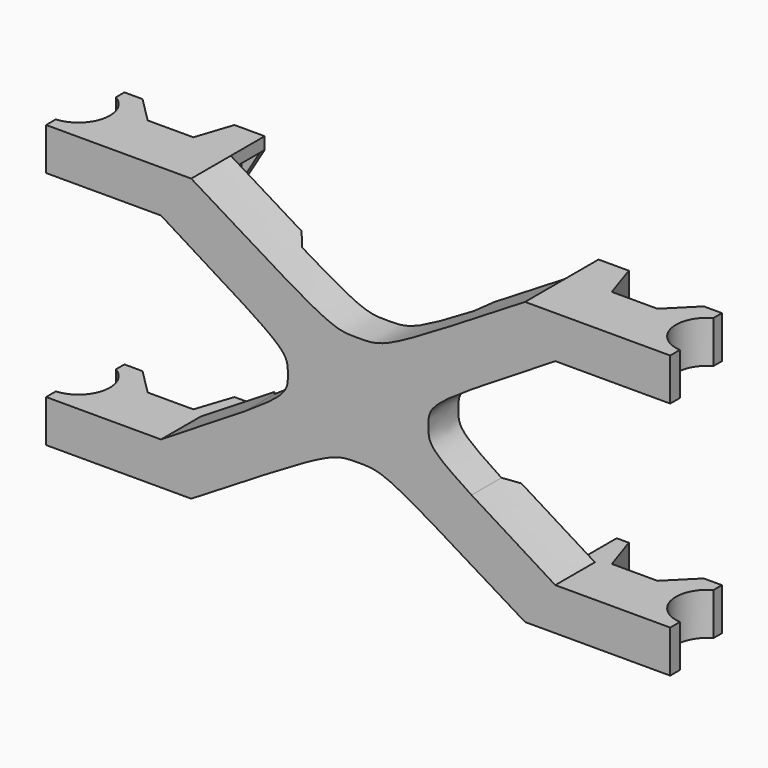
from build123d import *

# Parameters (mm, degrees)
F3_DEPTH = 25
F4_DEPTH = 15
F5_DEPTH = 3.5
F6_DEPTH = 4.5
F7_SIZE  = 0.99999
F8_DEPTH = 0.5


# Not quite as in the source:
# - a fillet or chamfer is up to 0.001 mm smaller than in the source, because OpenCascade refuses the exact size


with BuildPart() as f3:
    # F1 (on Front) → F3 (new body)
    with BuildSketch(Plane.XZ):
        Polygon((-13.8, 10.65), (-13.8, 11.65), (-27.9639077127, 11.65), (-27.9639077127, 8.15), (-16.3, 8.15), (-15.3, 8.15), (-15.3, 10.65), align=None)
        Polygon((-15.3, 8.15), (-13.8, 10.65), (-15.3, 10.65), align=None)
        with BuildLine():
            add(Edge.make_bspline(
                [(-13.8, 11.65), (-10.9198868997, 9.8796682436), (-8.756331306, 8.5497860338), (-7.0968113587, 7.5507717612)],
                knots=[0, 0, 0, 0, 3.862913837, 3.862913837, 3.862913837, 3.862913837], degree=3))
            Line((-13.8, 11.65), (-13.8, 10.65))
            Line((-13.8, 10.65), (-15.3, 8.15))
            Line((-15.3, 8.15), (-16.3, 8.15))
            add(Edge.make_bspline(
                [(-16.3, 8.15), (-13.129513862, 6.2011833744), (-10.9174831538, 4.8415047533), (-9.3741615176, 3.8458017731)],
                knots=[0, 0, 0, 0, 4.015251308, 4.015251308, 4.015251308, 4.015251308], degree=3))
            Line((-9.3741615176, 3.8458017731), (-7.0968113587, 7.5507717612))
        make_face()
        with BuildLine():
            add(Edge.make_bspline(
                [(-7.0968113587, 7.5507717612), (-2.0860988453, 4.5343733594), (-1.6704895359, 4.5343733594), (0, 4.5343733594)],
                knots=[3.862913837, 3.862913837, 3.862913837, 3.862913837, 15.5264980755, 15.5264980755, 15.5264980755, 15.5264980755], degree=3))
            Line((-7.0968113587, 7.5507717612), (-9.3741615176, 3.8458017731))
            add(Edge.make_bspline(
                [(-9.3741615176, 3.8458017731), (-5.812311122, 1.5478069994), (-5.812311122, 1.1885129773), (-5.812311122, 0)],
                knots=[4.015251308, 4.015251308, 4.015251308, 4.015251308, 13.2820976506, 13.2820976506, 13.2820976506, 13.2820976506], degree=3))
            add(Edge.make_bspline(
                [(-9.3741615176, -3.8458017731), (-5.812311122, -1.5478069994), (-5.812311122, -1.1885129773), (-5.812311122, 0)],
                knots=[4.015251308, 4.015251308, 4.015251308, 4.015251308, 13.2820976506, 13.2820976506, 13.2820976506, 13.2820976506], degree=3))
            Line((-9.3741615176, -3.8458017731), (-7.0968113587, -7.5507717612))
            add(Edge.make_bspline(
                [(-7.0968113587, -7.5507717612), (-2.0860988453, -4.5343733594), (-1.6704895359, -4.5343733594), (0, -4.5343733594)],
                knots=[3.862913837, 3.862913837, 3.862913837, 3.862913837, 15.5264980755, 15.5264980755, 15.5264980755, 15.5264980755], degree=3))
            add(Edge.make_bspline(
                [(7.0968113587, -7.5507717612), (2.0860988453, -4.5343733594), (1.6704895359, -4.5343733594), (0, -4.5343733594)],
                knots=[3.862913837, 3.862913837, 3.862913837, 3.862913837, 15.5264980755, 15.5264980755, 15.5264980755, 15.5264980755], degree=3))
            Line((7.0968113587, -7.5507717612), (9.3741615176, -3.8458017731))
            add(Edge.make_bspline(
                [(9.3741615176, -3.8458017731), (5.812311122, -1.5478069994), (5.812311122, -1.1885129773), (5.812311122, 0)],
                knots=[4.015251308, 4.015251308, 4.015251308, 4.015251308, 13.2820976506, 13.2820976506, 13.2820976506, 13.2820976506], degree=3))
            add(Edge.make_bspline(
                [(9.3741615176, 3.8458017731), (5.812311122, 1.5478069994), (5.812311122, 1.1885129773), (5.812311122, 0)],
                knots=[4.015251308, 4.015251308, 4.015251308, 4.015251308, 13.2820976506, 13.2820976506, 13.2820976506, 13.2820976506], degree=3))
            Line((9.3741615176, 3.8458017731), (7.0968113587, 7.5507717612))
            add(Edge.make_bspline(
                [(7.0968113587, 7.5507717612), (2.0860988453, 4.5343733594), (1.6704895359, 4.5343733594), (0, 4.5343733594)],
                knots=[3.862913837, 3.862913837, 3.862913837, 3.862913837, 15.5264980755, 15.5264980755, 15.5264980755, 15.5264980755], degree=3))
        make_face()
        with BuildLine():
            Line((-7.0968113587, -7.5507717612), (-9.3741615176, -3.8458017731))
            add(Edge.make_bspline(
                [(-16.3, -8.15), (-13.129513862, -6.2011833744), (-10.9174831538, -4.8415047533), (-9.3741615176, -3.8458017731)],
                knots=[0, 0, 0, 0, 4.015251308, 4.015251308, 4.015251308, 4.015251308], degree=3))
            Line((-16.3, -8.15), (-15.3, -8.15))
            Line((-15.3, -8.15), (-13.8, -10.65))
            Line((-13.8, -10.65), (-13.8, -11.65))
            add(Edge.make_bspline(
                [(-13.8, -11.65), (-10.9198868997, -9.8796682436), (-8.756331306, -8.5497860338), (-7.0968113587, -7.5507717612)],
                knots=[0, 0, 0, 0, 3.862913837, 3.862913837, 3.862913837, 3.862913837], degree=3))
        make_face()
        Polygon((-13.8, -10.65), (-15.3, -8.15), (-15.3, -10.65), align=None)
        Polygon((-15.3, -8.15), (-16.3, -8.15), (-27.9639077127, -8.15), (-27.9639077127, -11.65), (-13.8, -11.65), (-13.8, -10.65), (-15.3, -10.65), align=None)
        with BuildLine():
            add(Edge.make_bspline(
                [(16.3, -8.15), (13.129513862, -6.2011833744), (10.9174831538, -4.8415047533), (9.3741615176, -3.8458017731)],
                knots=[0, 0, 0, 0, 4.015251308, 4.015251308, 4.015251308, 4.015251308], degree=3))
            Line((9.3741615176, -3.8458017731), (7.0968113587, -7.5507717612))
            add(Edge.make_bspline(
                [(13.8, -11.65), (10.9198868997, -9.8796682436), (8.756331306, -8.5497860338), (7.0968113587, -7.5507717612)],
                knots=[0, 0, 0, 0, 3.862913837, 3.862913837, 3.862913837, 3.862913837], degree=3))
            Line((13.8, -11.65), (13.8, -10.65))
            Line((13.8, -10.65), (15.3, -8.15))
            Line((15.3, -8.15), (16.3, -8.15))
        make_face()
        Polygon((15.3, -10.65), (15.3, -8.15), (13.8, -10.65), align=None)
        Polygon((27.9639077127, -8.15), (16.3, -8.15), (15.3, -8.15), (15.3, -10.65), (13.8, -10.65), (13.8, -11.65), (27.9639077127, -11.65), align=None)
        with BuildLine():
            add(Edge.make_bspline(
                [(13.8, 11.65), (10.9198868997, 9.8796682436), (8.756331306, 8.5497860338), (7.0968113587, 7.5507717612)],
                knots=[0, 0, 0, 0, 3.862913837, 3.862913837, 3.862913837, 3.862913837], degree=3))
            Line((7.0968113587, 7.5507717612), (9.3741615176, 3.8458017731))
            add(Edge.make_bspline(
                [(16.3, 8.15), (13.129513862, 6.2011833744), (10.9174831538, 4.8415047533), (9.3741615176, 3.8458017731)],
                knots=[0, 0, 0, 0, 4.015251308, 4.015251308, 4.015251308, 4.015251308], degree=3))
            Line((16.3, 8.15), (15.3, 8.15))
            Line((15.3, 8.15), (13.8, 10.65))
            Line((13.8, 10.65), (13.8, 11.65))
        make_face()
        Polygon((27.9639077127, 11.65), (13.8, 11.65), (13.8, 10.65), (15.3, 10.65), (15.3, 8.15), (16.3, 8.15), (27.9639077127, 8.15), align=None)
        Polygon((15.3, 10.65), (13.8, 10.65), (15.3, 8.15), align=None)
    extrude(amount=F3_DEPTH)

    # F2 (on Top) → F4 (intersect, symmetric)
    with BuildSketch(Plane.XY):
        with BuildLine():
            Line((16.3, 0), (0, 0))
            Line((0, 0), (-16.3, 0))
            Line((-16.3, 0), (-17.3, -3))
            Line((-17.3, -3), (-21.0741669751, -3))
            Line((-21.0741669751, -3), (-23.2, -0.8741669751))
            Line((-23.2, -0.8741669751), (-24.7, -0.8741669751))
            Line((-24.7, -0.8741669751), (-24.7, -1.7483339502))
            ThreePointArc((-24.7, -1.7483339502), (-23.4645527492, -4.5757666527), (-25.8, -6.5922962794))
            Line((-25.8, -6.5922962794), (-25.8, -7.5922962794))
            Line((-25.8, -7.5922962794), (0, -7.5922962794))
            Line((0, -7.5922962794), (25.8, -7.5922962794))
            Line((25.8, -7.5922962794), (25.8, -6.5922962794))
            ThreePointArc((25.8, -6.5922962794), (23.4645527492, -4.5757666527), (24.7, -1.7483339502))
            Line((24.7, -1.7483339502), (24.7, -0.8741669751))
            Line((24.7, -0.8741669751), (23.2, -0.8741669751))
            Line((23.2, -0.8741669751), (21.0741669751, -3))
            Line((21.0741669751, -3), (17.3, -3))
            Line((17.3, -3), (16.3, 0))
        make_face()
    extrude(amount=F4_DEPTH, both=True, mode=Mode.INTERSECT)

    # F1 (on Front) → F5 (cut)
    with BuildSketch(Plane.XZ):
        with BuildLine():
            add(Edge.make_bspline(
                [(-13.8, 11.65), (-10.9198868997, 9.8796682436), (-8.756331306, 8.5497860338), (-7.0968113587, 7.5507717612)],
                knots=[0, 0, 0, 0, 3.862913837, 3.862913837, 3.862913837, 3.862913837], degree=3))
            Line((-13.8, 11.65), (-13.8, 10.65))
            Line((-13.8, 10.65), (-15.3, 8.15))
            Line((-15.3, 8.15), (-16.3, 8.15))
            add(Edge.make_bspline(
                [(-16.3, 8.15), (-13.129513862, 6.2011833744), (-10.9174831538, 4.8415047533), (-9.3741615176, 3.8458017731)],
                knots=[0, 0, 0, 0, 4.015251308, 4.015251308, 4.015251308, 4.015251308], degree=3))
            Line((-9.3741615176, 3.8458017731), (-7.0968113587, 7.5507717612))
        make_face()
        with BuildLine():
            add(Edge.make_bspline(
                [(-7.0968113587, 7.5507717612), (-2.0860988453, 4.5343733594), (-1.6704895359, 4.5343733594), (0, 4.5343733594)],
                knots=[3.862913837, 3.862913837, 3.862913837, 3.862913837, 15.5264980755, 15.5264980755, 15.5264980755, 15.5264980755], degree=3))
            Line((-7.0968113587, 7.5507717612), (-9.3741615176, 3.8458017731))
            add(Edge.make_bspline(
                [(-9.3741615176, 3.8458017731), (-5.812311122, 1.5478069994), (-5.812311122, 1.1885129773), (-5.812311122, 0)],
                knots=[4.015251308, 4.015251308, 4.015251308, 4.015251308, 13.2820976506, 13.2820976506, 13.2820976506, 13.2820976506], degree=3))
            add(Edge.make_bspline(
                [(-9.3741615176, -3.8458017731), (-5.812311122, -1.5478069994), (-5.812311122, -1.1885129773), (-5.812311122, 0)],
                knots=[4.015251308, 4.015251308, 4.015251308, 4.015251308, 13.2820976506, 13.2820976506, 13.2820976506, 13.2820976506], degree=3))
            Line((-9.3741615176, -3.8458017731), (-7.0968113587, -7.5507717612))
            add(Edge.make_bspline(
                [(-7.0968113587, -7.5507717612), (-2.0860988453, -4.5343733594), (-1.6704895359, -4.5343733594), (0, -4.5343733594)],
                knots=[3.862913837, 3.862913837, 3.862913837, 3.862913837, 15.5264980755, 15.5264980755, 15.5264980755, 15.5264980755], degree=3))
            add(Edge.make_bspline(
                [(7.0968113587, -7.5507717612), (2.0860988453, -4.5343733594), (1.6704895359, -4.5343733594), (0, -4.5343733594)],
                knots=[3.862913837, 3.862913837, 3.862913837, 3.862913837, 15.5264980755, 15.5264980755, 15.5264980755, 15.5264980755], degree=3))
            Line((7.0968113587, -7.5507717612), (9.3741615176, -3.8458017731))
            add(Edge.make_bspline(
                [(9.3741615176, -3.8458017731), (5.812311122, -1.5478069994), (5.812311122, -1.1885129773), (5.812311122, 0)],
                knots=[4.015251308, 4.015251308, 4.015251308, 4.015251308, 13.2820976506, 13.2820976506, 13.2820976506, 13.2820976506], degree=3))
            add(Edge.make_bspline(
                [(9.3741615176, 3.8458017731), (5.812311122, 1.5478069994), (5.812311122, 1.1885129773), (5.812311122, 0)],
                knots=[4.015251308, 4.015251308, 4.015251308, 4.015251308, 13.2820976506, 13.2820976506, 13.2820976506, 13.2820976506], degree=3))
            Line((9.3741615176, 3.8458017731), (7.0968113587, 7.5507717612))
            add(Edge.make_bspline(
                [(7.0968113587, 7.5507717612), (2.0860988453, 4.5343733594), (1.6704895359, 4.5343733594), (0, 4.5343733594)],
                knots=[3.862913837, 3.862913837, 3.862913837, 3.862913837, 15.5264980755, 15.5264980755, 15.5264980755, 15.5264980755], degree=3))
        make_face()
        with BuildLine():
            Line((-7.0968113587, -7.5507717612), (-9.3741615176, -3.8458017731))
            add(Edge.make_bspline(
                [(-16.3, -8.15), (-13.129513862, -6.2011833744), (-10.9174831538, -4.8415047533), (-9.3741615176, -3.8458017731)],
                knots=[0, 0, 0, 0, 4.015251308, 4.015251308, 4.015251308, 4.015251308], degree=3))
            Line((-16.3, -8.15), (-15.3, -8.15))
            Line((-15.3, -8.15), (-13.8, -10.65))
            Line((-13.8, -10.65), (-13.8, -11.65))
            add(Edge.make_bspline(
                [(-13.8, -11.65), (-10.9198868997, -9.8796682436), (-8.756331306, -8.5497860338), (-7.0968113587, -7.5507717612)],
                knots=[0, 0, 0, 0, 3.862913837, 3.862913837, 3.862913837, 3.862913837], degree=3))
        make_face()
        with BuildLine():
            add(Edge.make_bspline(
                [(16.3, -8.15), (13.129513862, -6.2011833744), (10.9174831538, -4.8415047533), (9.3741615176, -3.8458017731)],
                knots=[0, 0, 0, 0, 4.015251308, 4.015251308, 4.015251308, 4.015251308], degree=3))
            Line((9.3741615176, -3.8458017731), (7.0968113587, -7.5507717612))
            add(Edge.make_bspline(
                [(13.8, -11.65), (10.9198868997, -9.8796682436), (8.756331306, -8.5497860338), (7.0968113587, -7.5507717612)],
                knots=[0, 0, 0, 0, 3.862913837, 3.862913837, 3.862913837, 3.862913837], degree=3))
            Line((13.8, -11.65), (13.8, -10.65))
            Line((13.8, -10.65), (15.3, -8.15))
            Line((15.3, -8.15), (16.3, -8.15))
        make_face()
        with BuildLine():
            add(Edge.make_bspline(
                [(13.8, 11.65), (10.9198868997, 9.8796682436), (8.756331306, 8.5497860338), (7.0968113587, 7.5507717612)],
                knots=[0, 0, 0, 0, 3.862913837, 3.862913837, 3.862913837, 3.862913837], degree=3))
            Line((7.0968113587, 7.5507717612), (9.3741615176, 3.8458017731))
            add(Edge.make_bspline(
                [(16.3, 8.15), (13.129513862, 6.2011833744), (10.9174831538, 4.8415047533), (9.3741615176, 3.8458017731)],
                knots=[0, 0, 0, 0, 4.015251308, 4.015251308, 4.015251308, 4.015251308], degree=3))
            Line((16.3, 8.15), (15.3, 8.15))
            Line((15.3, 8.15), (13.8, 10.65))
            Line((13.8, 10.65), (13.8, 11.65))
        make_face()
        Polygon((-15.3, 8.15), (-13.8, 10.65), (-15.3, 10.65), align=None)
        Polygon((-13.8, -10.65), (-15.3, -8.15), (-15.3, -10.65), align=None)
        Polygon((15.3, -10.65), (15.3, -8.15), (13.8, -10.65), align=None)
        Polygon((15.3, 10.65), (13.8, 10.65), (15.3, 8.15), align=None)
    extrude(amount=F5_DEPTH, mode=Mode.SUBTRACT)

    # F1 (on Front) → F6 (cut)
    with BuildSketch(Plane.XZ):
        with BuildLine():
            add(Edge.make_bspline(
                [(-7.0968113587, 7.5507717612), (-2.0860988453, 4.5343733594), (-1.6704895359, 4.5343733594), (0, 4.5343733594)],
                knots=[3.862913837, 3.862913837, 3.862913837, 3.862913837, 15.5264980755, 15.5264980755, 15.5264980755, 15.5264980755], degree=3))
            Line((-7.0968113587, 7.5507717612), (-9.3741615176, 3.8458017731))
            add(Edge.make_bspline(
                [(-9.3741615176, 3.8458017731), (-5.812311122, 1.5478069994), (-5.812311122, 1.1885129773), (-5.812311122, 0)],
                knots=[4.015251308, 4.015251308, 4.015251308, 4.015251308, 13.2820976506, 13.2820976506, 13.2820976506, 13.2820976506], degree=3))
            add(Edge.make_bspline(
                [(-9.3741615176, -3.8458017731), (-5.812311122, -1.5478069994), (-5.812311122, -1.1885129773), (-5.812311122, 0)],
                knots=[4.015251308, 4.015251308, 4.015251308, 4.015251308, 13.2820976506, 13.2820976506, 13.2820976506, 13.2820976506], degree=3))
            Line((-9.3741615176, -3.8458017731), (-7.0968113587, -7.5507717612))
            add(Edge.make_bspline(
                [(-7.0968113587, -7.5507717612), (-2.0860988453, -4.5343733594), (-1.6704895359, -4.5343733594), (0, -4.5343733594)],
                knots=[3.862913837, 3.862913837, 3.862913837, 3.862913837, 15.5264980755, 15.5264980755, 15.5264980755, 15.5264980755], degree=3))
            add(Edge.make_bspline(
                [(7.0968113587, -7.5507717612), (2.0860988453, -4.5343733594), (1.6704895359, -4.5343733594), (0, -4.5343733594)],
                knots=[3.862913837, 3.862913837, 3.862913837, 3.862913837, 15.5264980755, 15.5264980755, 15.5264980755, 15.5264980755], degree=3))
            Line((7.0968113587, -7.5507717612), (9.3741615176, -3.8458017731))
            add(Edge.make_bspline(
                [(9.3741615176, -3.8458017731), (5.812311122, -1.5478069994), (5.812311122, -1.1885129773), (5.812311122, 0)],
                knots=[4.015251308, 4.015251308, 4.015251308, 4.015251308, 13.2820976506, 13.2820976506, 13.2820976506, 13.2820976506], degree=3))
            add(Edge.make_bspline(
                [(9.3741615176, 3.8458017731), (5.812311122, 1.5478069994), (5.812311122, 1.1885129773), (5.812311122, 0)],
                knots=[4.015251308, 4.015251308, 4.015251308, 4.015251308, 13.2820976506, 13.2820976506, 13.2820976506, 13.2820976506], degree=3))
            Line((9.3741615176, 3.8458017731), (7.0968113587, 7.5507717612))
            add(Edge.make_bspline(
                [(7.0968113587, 7.5507717612), (2.0860988453, 4.5343733594), (1.6704895359, 4.5343733594), (0, 4.5343733594)],
                knots=[3.862913837, 3.862913837, 3.862913837, 3.862913837, 15.5264980755, 15.5264980755, 15.5264980755, 15.5264980755], degree=3))
        make_face()
    extrude(amount=F6_DEPTH, mode=Mode.SUBTRACT)

    # F7 (size 1 in the source; OpenCascade refuses exactly that, so slightly less here)
    f7_edges = [f3.edges().sort_by_distance(p)[0] for p in [
        (8.235486, -3.5, 5.698287),
        (-8.235486, -3.5, 5.698287),
        (-8.235486, -3.5, -5.698287),
        (8.235486, -3.5, -5.698287),
    ]]
    chamfer(f7_edges, length=F7_SIZE)

    # F1 (on Front) → F8 (join)
    with BuildSketch(Plane.XZ):
        Polygon((15.3, -10.65), (15.3, -8.15), (13.8, -10.65), align=None)
        Polygon((-13.8, -10.65), (-15.3, -8.15), (-15.3, -10.65), align=None)
        Polygon((-15.3, 8.15), (-13.8, 10.65), (-15.3, 10.65), align=None)
    extrude(amount=F8_DEPTH)


solid = f3.part
